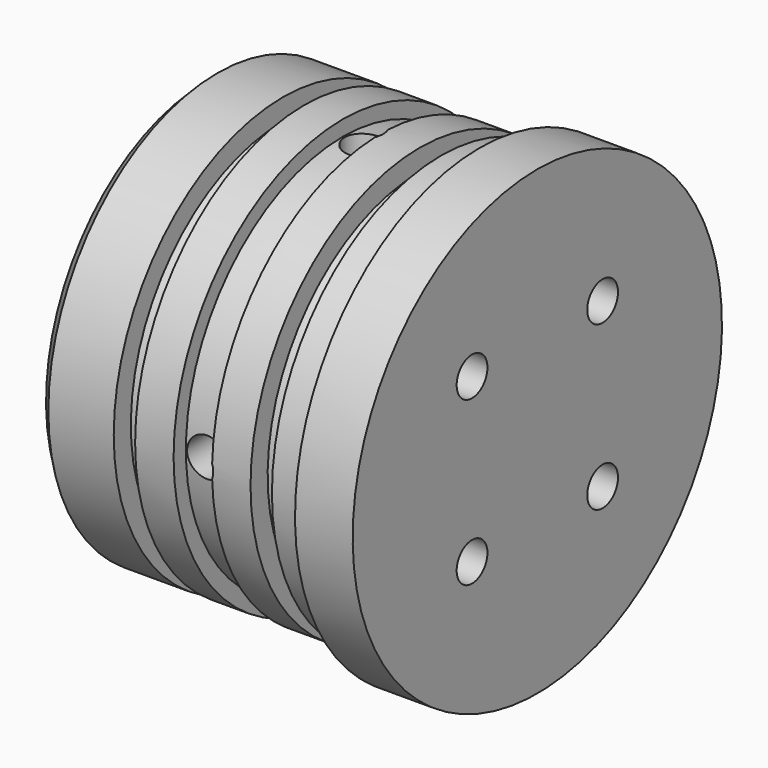
from build123d import *

# Parameters (mm, degrees)
F2_R      = 3.175
F3_DEPTH  = 38.1
F4_R      = 3.175
F5_DEPTH  = 38.1
F7_DEPTH  = 6.35
F8_SIZE   = 1.905
F9_R      = 3.175
F10_DEPTH = 9.525


# Not quite as in the source:
# - a feature names something its author has since deleted; it is built from what else it names


with BuildPart() as f1:
    # F0 (on Front) → F1 (revolve)
    with BuildSketch(Plane.XZ):
        Polygon((41.9862, 25.4), (41.9862, 0), (48.3362, 0), (48.3362, 25.527), (48.3362, 38.1), (45.1612, 38.1), (45.1612, 34.925), (38.8112, 34.925), (38.8112, 31.3944), (35.2806, 31.3944), (35.2806, 34.925), (28.9306, 34.925), (28.9306, 32.385), (22.5806, 32.385), (22.5806, 34.925), (16.2306, 34.925), (16.2306, 31.3944), (12.7, 31.3944), (12.7, 34.925), (0, 34.925), (0, 25.4), (5.08, 25.4), (5.08, 28.9306), (8.6106, 28.9306), (8.6106, 25.4), align=None)
    revolve(axis=Axis((-0.433858484, 0, 0), (1, 0, 0)))

    # F2 (on Front) → F3 (cut, symmetric)
    with BuildSketch(Plane.XZ):
        with Locations((25.9468089789, 0)):
            Circle(F2_R)
    extrude(amount=F3_DEPTH, both=True, mode=Mode.SUBTRACT)

    # F4 (on Top) → F5 (cut, symmetric)
    with BuildSketch(Plane.XY):
        with Locations((26.0544512421, 0)):
            Circle(F4_R)
    extrude(amount=F5_DEPTH, both=True, mode=Mode.SUBTRACT)

    # F7 (add): a face of the model
    f7_faces = [f1.faces().sort_by_distance(p)[0] for p in [
        (48.3362, 0, 0),
    ]]
    extrude(f7_faces, amount=F7_DEPTH)

    # F8
    f8_edges = [f1.edges().sort_by_distance(p)[0] for p in [
        (0, 0, -34.925),
    ]]
    chamfer(f8_edges, length=F8_SIZE)

    # F9 (on face) → F10 (cut)
    with BuildSketch(Plane.YZ.offset(54.6862)):
        with Locations((13.4703841816, 13.4703841816)):
            Circle(F9_R)
        with Locations((13.4703841816, -13.4703841816)):
            Circle(F9_R)
        with Locations((-13.4703841816, -13.4703841816)):
            Circle(F9_R)
        with Locations((-13.4703841816, 13.4703841816)):
            Circle(F9_R)
    extrude(amount=-F10_DEPTH, mode=Mode.SUBTRACT)


solid = f1.part
